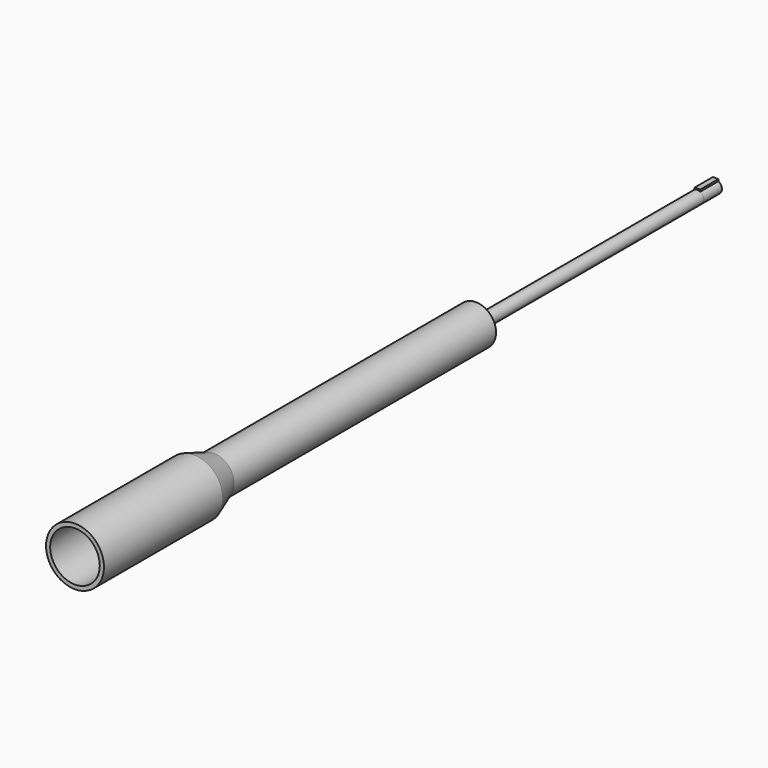
from build123d import *
from build123d import SkipClean  # not in build123d's __all__

# Parameters (mm, degrees)
F0_R      = 3
F0_R_2    = 2.275
F1_DEPTH  = 5
F5_R      = 1.25
F3_R      = 3
F7_DEPTH  = 110
F12_DEPTH = 4.5
F13_R     = 4
F13_R_2   = 3.3
F14_DEPTH = 60
F16_R     = 1.75
F18_R     = 4
F20_R     = 1.65
F21_DEPTH = 5
F23_R     = 4
F24_DEPTH = 5
F28_R     = 4
F27_R     = 5.75
F30_R     = 3.75
F31_R     = 4.925
F33_DEPTH = 29.5
F34_DEPTH = 29.6


# Not quite as in the source:
# - after a boolean that leaves OpenCascade's solid faulty, fix() repairs it


with BuildPart() as f1:
    # F0 (on Front) → F1 (new body)
    with BuildSketch(Plane.XZ):
        Circle(F0_R)
        Circle(F0_R_2, mode=Mode.SUBTRACT)
    extrude(amount=-F1_DEPTH)

    # F5 (on offset) → F6 section 0
    with BuildSketch(Plane.XZ.offset(-10)):
        Circle(F5_R)
    # F3 (on offset) → F6 section 1
    with BuildSketch(Plane.XZ.offset(-5)):
        Circle(F3_R)
    loft()

    # F5 (on offset) → F7 (join)
    with BuildSketch(Plane.XZ.offset(-10)):
        Circle(F5_R)
    extrude(amount=-F7_DEPTH)

    # F9 (on offset) → F12 (join)
    with BuildSketch(Plane.XZ.offset(-120)):
        with BuildLine():
            Line((-0.55, 1.5026115235), (-0.55, 1.122497216))
            ThreePointArc((-0.55, 1.122497216), (0, -1.25), (0.55, 1.122497216))
            Line((0.55, 1.122497216), (0.55, 1.5026115235))
            Line((0.55, 1.5026115235), (-0.55, 1.5026115235))
        make_face()
    extrude(amount=-F12_DEPTH)


with BuildPart() as f14:
    # F13 (on Front) → F14 (new body)
    with BuildSketch(Plane.XZ):
        Circle(F13_R)
        Circle(F13_R_2, mode=Mode.SUBTRACT)
    extrude(amount=-F14_DEPTH)

    # F16 (on offset) → F19 section 0
    with BuildSketch(Plane.XZ.offset(-57)):
        Circle(F16_R)
    # F18 (on offset) → F19 section 1
    with BuildSketch(Plane.XZ.offset(-55)):
        Circle(F18_R)
    loft()

    # F20 (on offset) → F21 (cut)
    with BuildSketch(Plane.XZ.offset(-55)):
        Circle(F20_R)
    extrude(amount=-F21_DEPTH, mode=Mode.SUBTRACT)

    # F23 (on offset) → F24 (join)
    with BuildSketch(Plane.XZ.offset(-60)):
        Circle(F23_R)
        with BuildLine():
            ThreePointArc((0.825, 3.1952112606), (0, -3.3), (-0.825, 3.1952112606))
            Line((-0.825, 3.1952112606), (-0.825, 3.6452112606))
            Line((-0.825, 3.6452112606), (0.825, 3.6452112606))
            Line((0.825, 3.6452112606), (0.825, 3.1952112606))
        make_face(mode=Mode.SUBTRACT)
    with SkipClean():  # cleaning this boolean's faces spoils the solid; the shape is the same uncleaned
        extrude(amount=-F24_DEPTH)

    # F28 (on Front) → F29 section 0
    with BuildSketch(Plane.XZ):
        Circle(F28_R)
    # F27 (on offset) → F29 section 1
    with BuildSketch(Plane.XZ.offset(5)):
        Circle(F27_R)
    loft()

    add(f14.part.fix(), mode=Mode.REPLACE)

    # F30 (on Front) → F32 section 0
    with BuildSketch(Plane.XZ):
        Circle(F30_R)
    # F31 (on offset) → F32 section 1
    with BuildSketch(Plane.XZ.offset(5)):
        Circle(F31_R)
    loft(mode=Mode.SUBTRACT)

    # F27 (on offset) → F33 (join)
    with BuildSketch(Plane.XZ.offset(5)):
        Circle(F27_R)
    extrude(amount=F33_DEPTH)

    # F31 (on offset) → F34 (cut)
    with BuildSketch(Plane.XZ.offset(5)):
        Circle(F31_R)
    extrude(amount=F34_DEPTH, mode=Mode.SUBTRACT)


solid = Compound([f1.part, f14.part])
